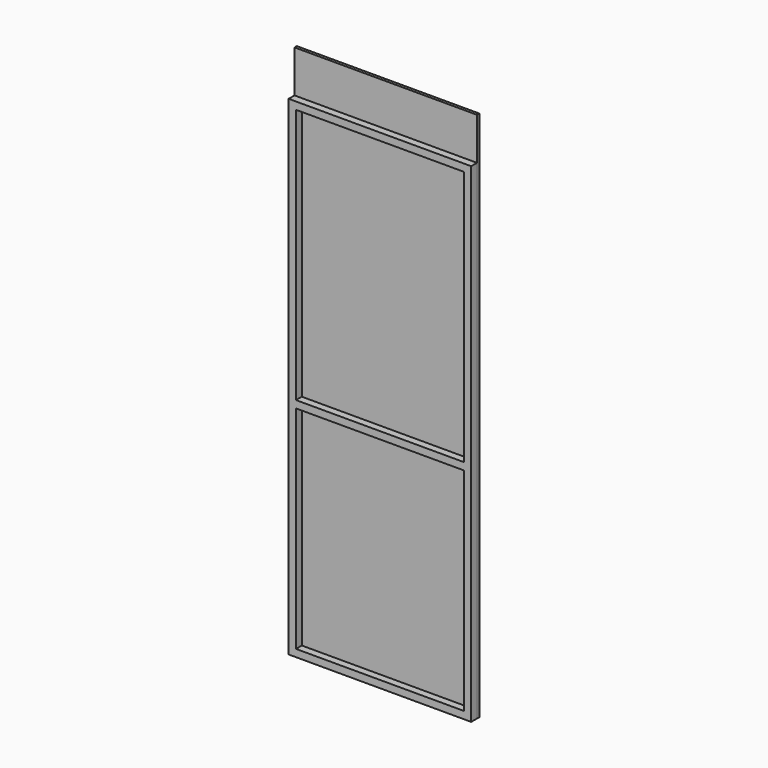
from build123d import *

# Parameters (mm, degrees)
F0_W     = 635
F0_H     = 1701.8
F1_DEPTH = 10.0076
F2_W     = 635
F2_H     = 1701.8
F2_W_2   = 584.2
F2_H_2   = 736.6
F2_H_3   = 889
F3_DEPTH = 25.4
F4_W     = 635
F4_H     = 10.0076
F5_DEPTH = 147.0152


with BuildPart() as f1:
    # F0 (on Front) → F1 (new body)
    with BuildSketch(Plane.XZ):
        with Locations((12.6779675484, 219.000581247)):
            Rectangle(F0_W, F0_H)
    extrude(amount=F1_DEPTH)

    # F4 (on face) → F5 (join)
    with BuildSketch(Plane.XY.offset(1069.900581247)):
        with Locations((12.6779675484, -5.0038)):
            Rectangle(F4_W, F4_H)
    extrude(amount=F5_DEPTH)


with BuildPart() as f3:
    # F2 (on face) → F3 (new body)
    with BuildSketch(Plane.XZ.offset(10.0076)):
        with Locations((12.6779675484, 219.000581247)):
            Rectangle(F2_W, F2_H)
        with Locations((12.6779675484, -238.199418753)):
            Rectangle(F2_W_2, F2_H_2, mode=Mode.SUBTRACT)
        with Locations((12.6779675484, 600.000581247)):
            Rectangle(F2_W_2, F2_H_3, mode=Mode.SUBTRACT)
    extrude(amount=F3_DEPTH)


solid = Compound([f1.part, f3.part])
